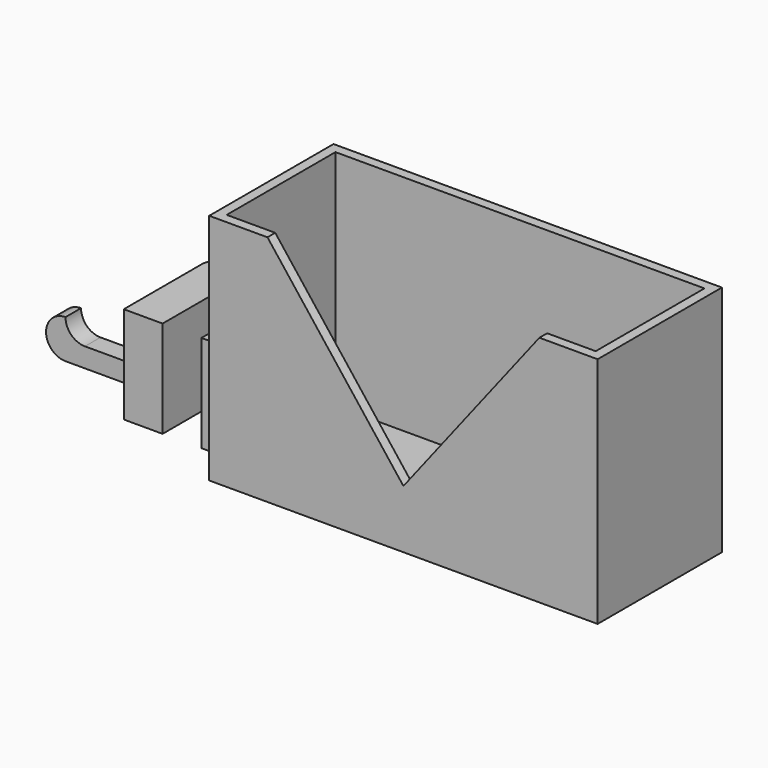
from build123d import *

# Parameters (mm, degrees)
F1_DEPTH  = 60
F2_T      = -2.5
F3_DEPTH  = 25
F4_W      = 25
F4_H      = 5
F5_DEPTH  = 5
F4_W_2    = 5
F6_DEPTH  = 10
F7_R      = 4.99999
F8_R      = 5
F10_DEPTH = 25


# Not quite as in the source:
# - a fillet or chamfer is up to 0.001 mm smaller than in the source, because OpenCascade refuses the exact size


with BuildPart() as f1:
    # F0 (on Top) → F1 (new body)
    with BuildSketch(Plane.XY):
        Polygon((0, 10), (0, 0), (100, 0), (100, 40), (0, 40), align=None)
    extrude(amount=F1_DEPTH)

    # F2
    f2_openings = [f1.faces().sort_by_distance(p)[0] for p in [
        (50, 20, 60),
    ]]
    offset(amount=F2_T, openings=f2_openings)

    # F9 (on face) → F10 (cut)
    with BuildSketch(Plane.XZ):
        Polygon((85, 60), (15, 60), (50, 15), align=None)
    extrude(amount=-F10_DEPTH, mode=Mode.SUBTRACT)


with BuildPart() as f3:
    # F0 (on Top) → F3 (new body)
    with BuildSketch(Plane.XY):
        Polygon((-10, 10), (0, 10), (0, 40), (-30, 40), (-30, 10), (-20, 10), (-20, 30), (-10, 30), align=None)
    extrude(amount=F3_DEPTH)

    # F4 (on Top) → F5 (join)
    with BuildSketch(Plane.XY):
        with Locations((-42.5, 25)):
            Rectangle(F4_W, F4_H)
    extrude(amount=F5_DEPTH)

    # F4 (on Top) → F6 (join)
    with BuildSketch(Plane.XY):
        with Locations((-57.5, 25)):
            Rectangle(F4_W_2, F4_H)
    extrude(amount=F6_DEPTH)

    # F7 (radius 5 in the source; OpenCascade refuses exactly that, so slightly less here)
    f7_edges = [f3.edges().sort_by_distance(p)[0] for p in [
        (-30, 25, 5),
        (-30, 22.5, 2.5),
        (-30, 27.5, 2.5),
        (-55, 25, 5),
        (-60, 25, 0),
        (-60, 25, 10),
    ]]
    fillet(f7_edges, radius=F7_R)

    # F8
    f8_edges = [f3.edges().sort_by_distance(p)[0] for p in [
        (-30, 40, 12.5),
    ]]
    fillet(f8_edges, radius=F8_R)


solid = Compound([f1.part, f3.part])
